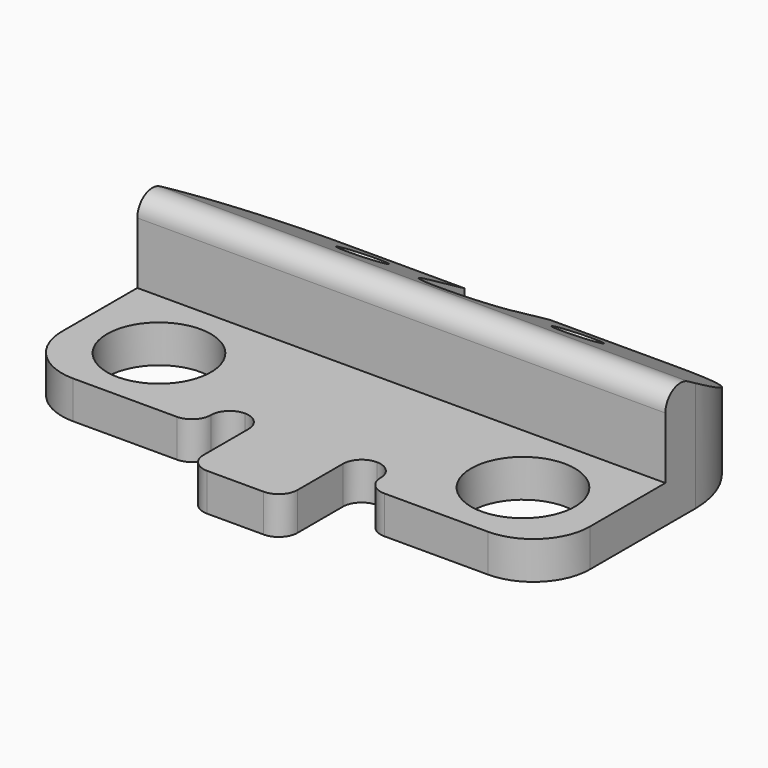
from build123d import *

# Parameters (mm, degrees)
F0_W      = 5
F0_H      = 3
F1_DEPTH  = 2
F0_W_2    = 28
F0_H_2    = 7
F2_DEPTH  = 7
F3_D      = 5.5
F5_DEPTH  = 28.001
F6_R      = 3
F7_R      = 5
F8_R      = 0.99999
F9_W      = 4.5
F9_H      = 3.1342408076
F10_DEPTH = 25
F11_D     = 2.3


# Not quite as in the source:
# - a fillet or chamfer is up to 0.001 mm smaller than in the source, because OpenCascade refuses the exact size


with BuildPart() as f1:
    # F0 (on Top) → F1 (new body)
    with BuildSketch(Plane.XY):
        Polygon((-14, -2), (-14, -10), (-4.5, -10), (-4.5, -8), (-2.5, -8), (-2.5, -10), (2.5, -10), (2.5, -8), (4.5, -8), (4.5, -10), (14, -10), (14, -2), align=None)
        with Locations((0, -11.5)):
            Rectangle(F0_W, F0_H)
    extrude(amount=F1_DEPTH)

    # F0 (on Top) → F2 (join)
    with BuildSketch(Plane.XY):
        with Locations((0, 1.5)):
            Rectangle(F0_W_2, F0_H_2)
    extrude(amount=F2_DEPTH)

    # F3 (through all)
    with Locations(Plane(origin=(0, 0, 0), x_dir=(1, 0, 0), z_dir=(0, 0, -1))):
        with Locations((-9.65, 6), (9.65, 6)):
            Hole(F3_D / 2)

    # F4 (on face) → F5 (cut, through all)
    with BuildSketch(Plane.YZ.offset(14)):
        Polygon((5, 7), (-2, 7), (5, 2.9585481157), align=None)
    extrude(amount=-F5_DEPTH, mode=Mode.SUBTRACT)

    # F6
    f6_edges = [f1.edges().sort_by_distance(p)[0] for p in [
        (-14, -10, 1),
        (14, -10, 1),
    ]]
    fillet(f6_edges, radius=F6_R)

    # F7
    f7_edges = [f1.edges().sort_by_distance(p)[0] for p in [
        (14, 5, 1.479274),
        (-14, 5, 1.479274),
    ]]
    fillet(f7_edges, radius=F7_R)

    # F8 (radius 1 in the source; OpenCascade refuses exactly that, so slightly less here)
    f8_edges = [f1.edges().sort_by_distance(p)[0] for p in [
        (0, -2, 7),
        (-4.5, -8, 1),
        (-2.5, -8, 1),
        (2.5, -8, 1),
        (4.5, -8, 1),
        (4.5, -10, 1),
        (-4.5, -10, 1),
        (-2.5, -13, 1),
        (2.5, -13, 1),
    ]]
    fillet(f8_edges, radius=F8_R)

    # F9 (on face) → F10 (cut)
    with BuildSketch(Plane(origin=(0, 2.5310889132, 4.3839745962), x_dir=(1, 0, 0), z_dir=(0, 0.5, 0.8660254038))):
        with BuildLine():
            Line((2.25, 2.8508529611), (-2.25, 2.8508529611))
            Line((-2.25, 2.8508529611), (-2.25, 0.0272258071))
            ThreePointArc((-2.25, 0.0272258071), (0, -2.2227741929), (2.25, 0.0272258071))
            Line((2.25, 0.0272258071), (2.25, 2.8508529611))
        make_face()
        with Locations((0, 4.4179733649)):
            Rectangle(F9_W, F9_H)
    extrude(amount=-F10_DEPTH, mode=Mode.SUBTRACT)

    # F11 (through all)
    with Locations(Plane(origin=(0, 2.5310889132, 4.3839745962), x_dir=(1, 0, 0), z_dir=(0, 0.5, 0.8660254038))):
        with Locations((5.7, 0.0272258071), (-5.7, 0.0272258071)):
            Hole(F11_D / 2)


solid = f1.part
